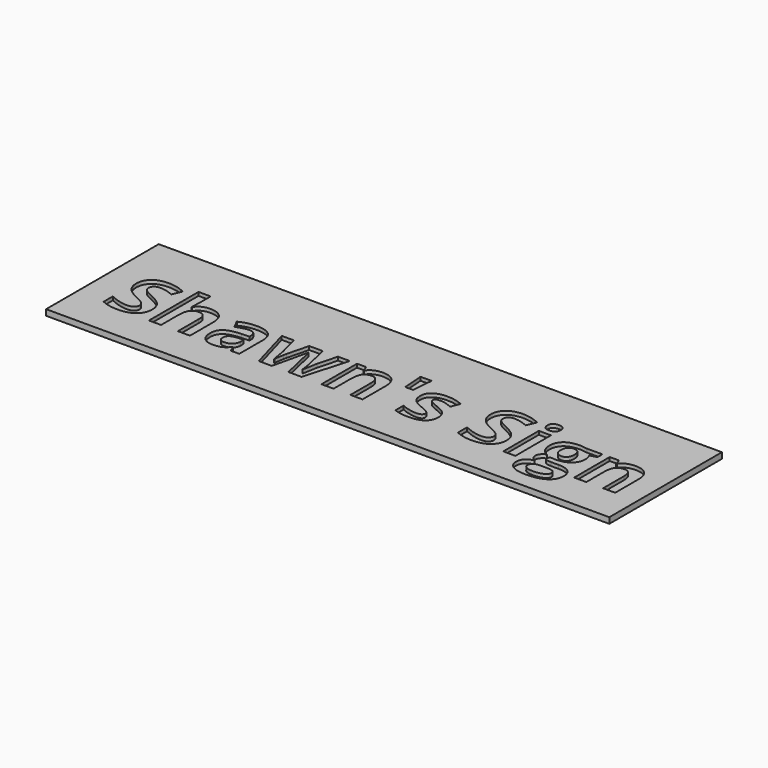
from build123d import *

# Parameters (mm, degrees)
F0_W         = 609.6
F0_H         = 152.4
F1_DEPTH     = 6.35
F2_TEXT_SIZE = 88.1944444444
F3_DEPTH     = 3.81


# Not quite as in the source:
# - Text() gives the source's letters only with a copy of the font that has no kerning and outlines rounded to 1/6400 em; it was checked with that copy


with BuildPart() as f1:
    # F0 (on Top) → F1 (new body)
    with BuildSketch(Plane.XY):
        with Locations((188.5758888503, -20.1630853117)):
            Rectangle(F0_W, F0_H)
    extrude(amount=F1_DEPTH)

    # F2 (on face) → F3 (cut)
    with BuildSketch(Plane.XY.offset(6.35)):
        with Locations((-90.8241111497, -58.2630853117)):
            Text("Shawn's Sign", F2_TEXT_SIZE, font='Open Sans', font_style=FontStyle.BOLD, text_align=(TextAlign.LEFT, TextAlign.BOTTOM))
    extrude(amount=-F3_DEPTH, mode=Mode.SUBTRACT)


solid = f1.part
